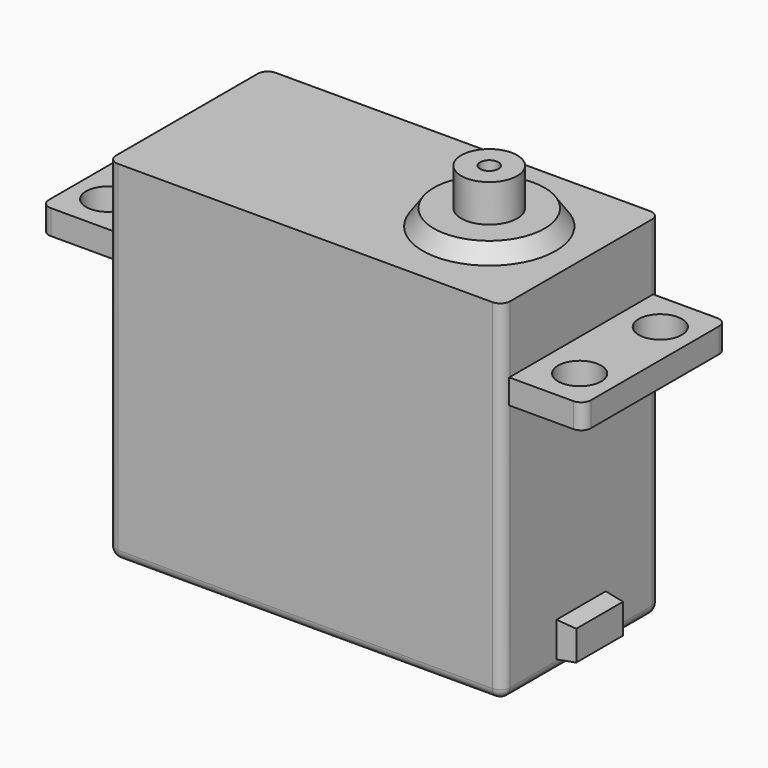
from build123d import *

# Parameters (mm, degrees)
F0_W           = 40.64
F0_H           = 20.32
F1_DEPTH       = 36.068
F2_W           = 6.35
F2_H           = 3.6068
F4_W           = 6.0198
F4_H           = 3.0734
F7_R           = 2.2225
F8_DEPTH       = 2.54
F9_R           = 6.858
F11_R          = 5.7023
F13_T1_DEPTH   = 38.608
F13_T3_DEPTH   = 18.288
F13_S7_W       = 1.016
F13_S7_H       = 1.016
F13_T8_DEPTH   = 1.016
F13_S13_W      = 1.016
F13_S13_H      = 1.016
F13_T14_DEPTH  = 1.016
F13_S19_W      = 1.016
F13_S19_H      = 1.016
F13_T20_DEPTH  = 1.016
F13_S25_W      = 1.016
F13_S25_H      = 1.016
F13_T26_DEPTH  = 1.016
F13_T32_DEPTH  = 37.592
F13_T38_DEPTH  = 37.592
F13_T44_DEPTH  = 37.592
F13_T51_DEPTH  = 37.592
F13_T57_DEPTH  = 37.592
F13_T63_DEPTH  = 37.592
F13_T69_DEPTH  = 37.592
F13_T75_DEPTH  = 37.592
F13_T82_DEPTH  = 37.592
F13_T88_DEPTH  = 37.592
F13_T94_DEPTH  = 37.592
F13_T100_DEPTH = 37.592
F13_T106_DEPTH = 37.592
F13_T113_DEPTH = 37.592
F13_T119_DEPTH = 37.592
F13_T125_DEPTH = 37.592
F13_T131_DEPTH = 37.592
F13_T137_DEPTH = 37.592
F13_T144_DEPTH = 37.592
F13_T150_DEPTH = 37.592
F14_R          = 2.8829
F14_R_2        = 0.9398
F15_DEPTH      = 3.8608


# Not quite as in the source:
# - a fillet or chamfer that OpenCascade refuses, or shapes differently, is made with other operations: its cross-section is extruded or revolved along the edge and cut away or added


with BuildPart() as f1:
    # F0 (on Top) → F1 (new body)
    with BuildSketch(Plane.XY):
        Rectangle(F0_W, F0_H)
    extrude(amount=F1_DEPTH)

    # F2 (on face) → F5 section 0
    with BuildSketch(Plane.YZ.offset(20.32)):
        with Locations((0, 2.9464)):
            Rectangle(F2_W, F2_H)
    # F4 (on offset) → F5 section 1
    with BuildSketch(Plane.YZ.offset(22.225)):
        with Locations((0, 2.9464)):
            Rectangle(F4_W, F4_H)
    loft()

    # F7 (on offset) → F8 (join)
    with BuildSketch(Plane.XY.offset(29.21)):
        with BuildLine():
            ThreePointArc((-27.94, -8.255), (-27.6424204897, -8.9734204897), (-26.924, -9.271))
            Line((-26.924, -9.271), (-20.32, -9.271))
            Line((-20.32, -9.271), (-20.32, 9.271))
            Line((-20.32, 9.271), (-26.924, 9.271))
            ThreePointArc((-26.924, 9.271), (-27.6424204897, 8.9734204897), (-27.94, 8.255))
            Line((-27.94, 8.255), (-27.94, -8.255))
        make_face()
        with Locations((-24.3205, -5.1943)):
            Circle(F7_R, mode=Mode.SUBTRACT)
        with Locations((-24.3205, 5.1943)):
            Circle(F7_R, mode=Mode.SUBTRACT)
        with BuildLine():
            ThreePointArc((27.94, 8.255), (27.6424204897, 8.9734204897), (26.924, 9.271))
            Line((26.924, 9.271), (20.32, 9.271))
            Line((20.32, 9.271), (20.32, -9.271))
            Line((20.32, -9.271), (26.924, -9.271))
            ThreePointArc((26.924, -9.271), (27.6424204897, -8.9734204897), (27.94, -8.255))
            Line((27.94, -8.255), (27.94, 8.255))
        make_face()
        with Locations((24.3205, -5.1943)):
            Circle(F7_R, mode=Mode.SUBTRACT)
        with Locations((24.3205, 5.1943)):
            Circle(F7_R, mode=Mode.SUBTRACT)
    extrude(amount=-F8_DEPTH)

    # F9 (on face) → F12 section 0
    with BuildSketch(Plane.XY.offset(36.068)):
        with Locations((10.8458, 0)):
            Circle(F9_R)
    # F11 (on offset) → F12 section 1
    with BuildSketch(Plane.XY.offset(37.719)):
        with Locations((10.8458, 0)):
            Circle(F11_R)
    loft()

    # F13: fillet of radius 1.016 on 8 edges, made by hand

    # F13_s2 → F13_t1 (cut)
    with BuildSketch(Plane.YZ.offset(-19.304)):
        with BuildLine():
            ThreePointArc((-10.16, 1.016), (-9.8624204897, 0.2975795103), (-9.144, 0))
            Line((-9.144, 0), (-10.16, 0))
            Line((-10.16, 0), (-10.16, 1.016))
        make_face()
        with BuildLine():
            ThreePointArc((9.144, 0), (9.8624204897, 0.2975795103), (10.16, 1.016))
            Line((10.16, 1.016), (10.16, 0))
            Line((10.16, 0), (9.144, 0))
        make_face()
    extrude(amount=F13_T1_DEPTH, mode=Mode.SUBTRACT)

    # F13_s4 → F13_t3 (cut)
    with BuildSketch(Plane.XZ.offset(-9.144)):
        with BuildLine():
            ThreePointArc((20.32, 1.016), (20.0224204897, 0.2975795103), (19.304, 0))
            Line((19.304, 0), (20.32, 0))
            Line((20.32, 0), (20.32, 1.016))
        make_face()
        with BuildLine():
            ThreePointArc((-19.304, 0), (-20.0224204897, 0.2975795103), (-20.32, 1.016))
            Line((-20.32, 1.016), (-20.32, 0))
            Line((-20.32, 0), (-19.304, 0))
        make_face()
    extrude(amount=F13_T3_DEPTH, mode=Mode.SUBTRACT)


with BuildPart() as f13_tool6:
    # F13_s7 → F13_t8 (new body)
    with BuildSketch(Plane.YZ.offset(19.304)):
        with Locations((-9.652, 0.508)):
            Rectangle(F13_S7_W, F13_S7_H)
    extrude(amount=F13_T8_DEPTH)

    # F13_s9 → F13_t10 (revolve, cut)
    with BuildSketch(Plane(origin=(19.304, -9.144, 1.016), x_dir=(0, 0.7071067812, 0.7071067812), z_dir=(0, 0.7071067812, -0.7071067812))):
        with BuildLine():
            ThreePointArc((0, -1.016), (1.016, 0), (0, 1.016))
            Line((0, 1.016), (0, -1.016))
        make_face()
    revolve(axis=Axis((19.304, -9.144, 1.016), (1, 0, 0)), mode=Mode.SUBTRACT)


with BuildPart() as f1_1:
    add(f1.part)

    # F13_t5: cut F13_tool6
    add(f13_tool6.part, mode=Mode.SUBTRACT)


with BuildPart() as f13_tool12:
    # F13_s13 → F13_t14 (new body)
    with BuildSketch(Plane.YZ.offset(19.304)):
        with Locations((9.652, 0.508)):
            Rectangle(F13_S13_W, F13_S13_H)
    extrude(amount=F13_T14_DEPTH)

    # F13_s15 → F13_t16 (revolve, cut)
    with BuildSketch(Plane(origin=(19.304, 9.144, 1.016), x_dir=(0, -0.7071067812, 0.7071067812), z_dir=(0, 0.7071067812, 0.7071067812))):
        with BuildLine():
            ThreePointArc((0, -1.016), (1.016, 0), (0, 1.016))
            Line((0, 1.016), (0, -1.016))
        make_face()
    revolve(axis=Axis((19.304, 9.144, 1.016), (1, 0, 0)), mode=Mode.SUBTRACT)


with BuildPart() as f1_2:
    add(f1_1.part)

    # F13_t11: cut F13_tool12
    add(f13_tool12.part, mode=Mode.SUBTRACT)


with BuildPart() as f13_tool18:
    # F13_s19 → F13_t20 (new body)
    with BuildSketch(Plane.XY.offset(1.016)):
        with Locations((-19.812, 9.652)):
            Rectangle(F13_S19_W, F13_S19_H)
    extrude(amount=-F13_T20_DEPTH)

    # F13_s21 → F13_t22 (revolve, cut)
    with BuildSketch(Plane(origin=(-19.304, 9.144, 1.016), x_dir=(0.7071067812, -0.7071067812, 0), z_dir=(0.7071067812, 0.7071067812, 0))):
        with BuildLine():
            ThreePointArc((0, -1.016), (1.016, 0), (0, 1.016))
            Line((0, 1.016), (0, -1.016))
        make_face()
    revolve(axis=Axis((-19.304, 9.144, 1.016), (0, 0, -1)), mode=Mode.SUBTRACT)


with BuildPart() as f1_3:
    add(f1_2.part)

    # F13_t17: cut F13_tool18
    add(f13_tool18.part, mode=Mode.SUBTRACT)


with BuildPart() as f13_tool24:
    # F13_s25 → F13_t26 (new body)
    with BuildSketch(Plane.XZ.offset(9.144)):
        with Locations((-19.812, 0.508)):
            Rectangle(F13_S25_W, F13_S25_H)
    extrude(amount=F13_T26_DEPTH)

    # F13_s27 → F13_t28 (revolve, cut)
    with BuildSketch(Plane(origin=(-19.304, -9.144, 1.016), x_dir=(0.7071067812, 0, 0.7071067812), z_dir=(0.7071067812, 0, -0.7071067812))):
        with BuildLine():
            ThreePointArc((0, -1.016), (1.016, 0), (0, 1.016))
            Line((0, 1.016), (0, -1.016))
        make_face()
    revolve(axis=Axis((-19.304, -9.144, 1.016), (0, -1, 0)), mode=Mode.SUBTRACT)


with BuildPart() as f1_4:
    add(f1_3.part)

    # F13_t23: cut F13_tool24
    add(f13_tool24.part, mode=Mode.SUBTRACT)


with BuildPart() as f13_tool30:
    # F13_s31 → F13_t32 (new body)
    with BuildSketch(Plane.XY.offset(1.016)):
        with BuildLine():
            ThreePointArc((20.32, -9.144), (20.0224204897, -9.8624204897), (19.304, -10.16))
            Line((19.304, -10.16), (20.32, -10.16))
            Line((20.32, -10.16), (20.32, -9.144))
        make_face()
    extrude(amount=F13_T32_DEPTH)

    split(bisect_by=Plane.XY.offset(26.67), keep=Keep.BOTTOM)

    split(bisect_by=Plane.XZ.offset(9.271), keep=Keep.BOTTOM)


with BuildPart() as f1_5:
    add(f1_4.part)

    # F13_t29: cut F13_tool30
    add(f13_tool30.part, mode=Mode.SUBTRACT)


with BuildPart() as f13_tool36:
    # F13_s37 → F13_t38 (new body)
    with BuildSketch(Plane.XY.offset(1.016)):
        with BuildLine():
            ThreePointArc((20.32, -9.144), (20.0224204897, -9.8624204897), (19.304, -10.16))
            Line((19.304, -10.16), (20.32, -10.16))
            Line((20.32, -10.16), (20.32, -9.144))
        make_face()
    extrude(amount=F13_T38_DEPTH)

    split(bisect_by=Plane.XY.offset(26.67), keep=Keep.BOTTOM)

    split(bisect_by=Plane.XZ.offset(9.271), keep=Keep.TOP)


with BuildPart() as f1_6:
    add(f1_5.part)

    # F13_t35: cut F13_tool36
    add(f13_tool36.part, mode=Mode.SUBTRACT)


with BuildPart() as f13_tool42:
    # F13_s43 → F13_t44 (new body)
    with BuildSketch(Plane.XY.offset(1.016)):
        with BuildLine():
            ThreePointArc((20.32, -9.144), (20.0224204897, -9.8624204897), (19.304, -10.16))
            Line((19.304, -10.16), (20.32, -10.16))
            Line((20.32, -10.16), (20.32, -9.144))
        make_face()
    extrude(amount=F13_T44_DEPTH)

    split(bisect_by=Plane.XY.offset(26.67), keep=Keep.TOP)

    split(bisect_by=Plane.XZ.offset(9.271), keep=Keep.TOP)

    split(bisect_by=Plane.XY.offset(29.21), keep=Keep.BOTTOM)


with BuildPart() as f1_7:
    add(f1_6.part)

    # F13_t41: cut F13_tool42
    add(f13_tool42.part, mode=Mode.SUBTRACT)


with BuildPart() as f13_tool49:
    # F13_s50 → F13_t51 (new body)
    with BuildSketch(Plane.XY.offset(1.016)):
        with BuildLine():
            ThreePointArc((20.32, -9.144), (20.0224204897, -9.8624204897), (19.304, -10.16))
            Line((19.304, -10.16), (20.32, -10.16))
            Line((20.32, -10.16), (20.32, -9.144))
        make_face()
    extrude(amount=F13_T51_DEPTH)

    split(bisect_by=Plane.XZ.offset(9.271), keep=Keep.BOTTOM)

    split(bisect_by=Plane.XY.offset(29.21), keep=Keep.TOP)


with BuildPart() as f1_8:
    add(f1_7.part)

    # F13_t48: cut F13_tool49
    add(f13_tool49.part, mode=Mode.SUBTRACT)


with BuildPart() as f13_tool55:
    # F13_s56 → F13_t57 (new body)
    with BuildSketch(Plane.XY.offset(1.016)):
        with BuildLine():
            ThreePointArc((20.32, -9.144), (20.0224204897, -9.8624204897), (19.304, -10.16))
            Line((19.304, -10.16), (20.32, -10.16))
            Line((20.32, -10.16), (20.32, -9.144))
        make_face()
    extrude(amount=F13_T57_DEPTH)

    split(bisect_by=Plane.XZ.offset(9.271), keep=Keep.TOP)

    split(bisect_by=Plane.XY.offset(29.21), keep=Keep.TOP)


with BuildPart() as f1_9:
    add(f1_8.part)

    # F13_t54: cut F13_tool55
    add(f13_tool55.part, mode=Mode.SUBTRACT)


with BuildPart() as f13_tool61:
    # F13_s62 → F13_t63 (new body)
    with BuildSketch(Plane.XY.offset(1.016)):
        with BuildLine():
            ThreePointArc((20.32, 9.144), (20.0224204897, 9.8624204897), (19.304, 10.16))
            Line((19.304, 10.16), (20.32, 10.16))
            Line((20.32, 10.16), (20.32, 9.144))
        make_face()
    extrude(amount=F13_T63_DEPTH)

    split(bisect_by=Plane.XZ.offset(-9.271), keep=Keep.TOP)

    split(bisect_by=Plane.XY.offset(26.67), keep=Keep.BOTTOM)


with BuildPart() as f1_10:
    add(f1_9.part)

    # F13_t60: cut F13_tool61
    add(f13_tool61.part, mode=Mode.SUBTRACT)


with BuildPart() as f13_tool67:
    # F13_s68 → F13_t69 (new body)
    with BuildSketch(Plane.XY.offset(1.016)):
        with BuildLine():
            ThreePointArc((20.32, 9.144), (20.0224204897, 9.8624204897), (19.304, 10.16))
            Line((19.304, 10.16), (20.32, 10.16))
            Line((20.32, 10.16), (20.32, 9.144))
        make_face()
    extrude(amount=F13_T69_DEPTH)

    split(bisect_by=Plane.XZ.offset(-9.271), keep=Keep.BOTTOM)

    split(bisect_by=Plane.XY.offset(26.67), keep=Keep.BOTTOM)


with BuildPart() as f1_11:
    add(f1_10.part)

    # F13_t66: cut F13_tool67
    add(f13_tool67.part, mode=Mode.SUBTRACT)


with BuildPart() as f13_tool73:
    # F13_s74 → F13_t75 (new body)
    with BuildSketch(Plane.XY.offset(1.016)):
        with BuildLine():
            ThreePointArc((20.32, 9.144), (20.0224204897, 9.8624204897), (19.304, 10.16))
            Line((19.304, 10.16), (20.32, 10.16))
            Line((20.32, 10.16), (20.32, 9.144))
        make_face()
    extrude(amount=F13_T75_DEPTH)

    split(bisect_by=Plane.XZ.offset(-9.271), keep=Keep.BOTTOM)

    split(bisect_by=Plane.XY.offset(26.67), keep=Keep.TOP)

    split(bisect_by=Plane.XY.offset(29.21), keep=Keep.BOTTOM)


with BuildPart() as f1_12:
    add(f1_11.part)

    # F13_t72: cut F13_tool73
    add(f13_tool73.part, mode=Mode.SUBTRACT)


with BuildPart() as f13_tool80:
    # F13_s81 → F13_t82 (new body)
    with BuildSketch(Plane.XY.offset(1.016)):
        with BuildLine():
            ThreePointArc((20.32, 9.144), (20.0224204897, 9.8624204897), (19.304, 10.16))
            Line((19.304, 10.16), (20.32, 10.16))
            Line((20.32, 10.16), (20.32, 9.144))
        make_face()
    extrude(amount=F13_T82_DEPTH)

    split(bisect_by=Plane.XZ.offset(-9.271), keep=Keep.TOP)

    split(bisect_by=Plane.XY.offset(29.21), keep=Keep.TOP)


with BuildPart() as f1_13:
    add(f1_12.part)

    # F13_t79: cut F13_tool80
    add(f13_tool80.part, mode=Mode.SUBTRACT)


with BuildPart() as f13_tool86:
    # F13_s87 → F13_t88 (new body)
    with BuildSketch(Plane.XY.offset(1.016)):
        with BuildLine():
            ThreePointArc((20.32, 9.144), (20.0224204897, 9.8624204897), (19.304, 10.16))
            Line((19.304, 10.16), (20.32, 10.16))
            Line((20.32, 10.16), (20.32, 9.144))
        make_face()
    extrude(amount=F13_T88_DEPTH)

    split(bisect_by=Plane.XZ.offset(-9.271), keep=Keep.BOTTOM)

    split(bisect_by=Plane.XY.offset(29.21), keep=Keep.TOP)


with BuildPart() as f1_14:
    add(f1_13.part)

    # F13_t85: cut F13_tool86
    add(f13_tool86.part, mode=Mode.SUBTRACT)


with BuildPart() as f13_tool92:
    # F13_s93 → F13_t94 (new body)
    with BuildSketch(Plane.XY.offset(1.016)):
        with BuildLine():
            ThreePointArc((-19.304, 10.16), (-20.0224204897, 9.8624204897), (-20.32, 9.144))
            Line((-20.32, 9.144), (-20.32, 10.16))
            Line((-20.32, 10.16), (-19.304, 10.16))
        make_face()
    extrude(amount=F13_T94_DEPTH)

    split(bisect_by=Plane.XY.offset(26.67), keep=Keep.BOTTOM)

    split(bisect_by=Plane.XZ.offset(-9.271), keep=Keep.BOTTOM)


with BuildPart() as f1_15:
    add(f1_14.part)

    # F13_t91: cut F13_tool92
    add(f13_tool92.part, mode=Mode.SUBTRACT)


with BuildPart() as f13_tool98:
    # F13_s99 → F13_t100 (new body)
    with BuildSketch(Plane.XY.offset(1.016)):
        with BuildLine():
            ThreePointArc((-19.304, 10.16), (-20.0224204897, 9.8624204897), (-20.32, 9.144))
            Line((-20.32, 9.144), (-20.32, 10.16))
            Line((-20.32, 10.16), (-19.304, 10.16))
        make_face()
    extrude(amount=F13_T100_DEPTH)

    split(bisect_by=Plane.XY.offset(26.67), keep=Keep.BOTTOM)

    split(bisect_by=Plane.XZ.offset(-9.271), keep=Keep.TOP)


with BuildPart() as f1_16:
    add(f1_15.part)

    # F13_t97: cut F13_tool98
    add(f13_tool98.part, mode=Mode.SUBTRACT)


with BuildPart() as f13_tool104:
    # F13_s105 → F13_t106 (new body)
    with BuildSketch(Plane.XY.offset(1.016)):
        with BuildLine():
            ThreePointArc((-19.304, 10.16), (-20.0224204897, 9.8624204897), (-20.32, 9.144))
            Line((-20.32, 9.144), (-20.32, 10.16))
            Line((-20.32, 10.16), (-19.304, 10.16))
        make_face()
    extrude(amount=F13_T106_DEPTH)

    split(bisect_by=Plane.XY.offset(26.67), keep=Keep.TOP)

    split(bisect_by=Plane.XZ.offset(-9.271), keep=Keep.BOTTOM)

    split(bisect_by=Plane.XY.offset(29.21), keep=Keep.BOTTOM)


with BuildPart() as f1_17:
    add(f1_16.part)

    # F13_t103: cut F13_tool104
    add(f13_tool104.part, mode=Mode.SUBTRACT)


with BuildPart() as f13_tool111:
    # F13_s112 → F13_t113 (new body)
    with BuildSketch(Plane.XY.offset(1.016)):
        with BuildLine():
            ThreePointArc((-19.304, 10.16), (-20.0224204897, 9.8624204897), (-20.32, 9.144))
            Line((-20.32, 9.144), (-20.32, 10.16))
            Line((-20.32, 10.16), (-19.304, 10.16))
        make_face()
    extrude(amount=F13_T113_DEPTH)

    split(bisect_by=Plane.XZ.offset(-9.271), keep=Keep.BOTTOM)

    split(bisect_by=Plane.XY.offset(29.21), keep=Keep.TOP)


with BuildPart() as f1_18:
    add(f1_17.part)

    # F13_t110: cut F13_tool111
    add(f13_tool111.part, mode=Mode.SUBTRACT)


with BuildPart() as f13_tool117:
    # F13_s118 → F13_t119 (new body)
    with BuildSketch(Plane.XY.offset(1.016)):
        with BuildLine():
            ThreePointArc((-19.304, 10.16), (-20.0224204897, 9.8624204897), (-20.32, 9.144))
            Line((-20.32, 9.144), (-20.32, 10.16))
            Line((-20.32, 10.16), (-19.304, 10.16))
        make_face()
    extrude(amount=F13_T119_DEPTH)

    split(bisect_by=Plane.XZ.offset(-9.271), keep=Keep.TOP)

    split(bisect_by=Plane.XY.offset(29.21), keep=Keep.TOP)


with BuildPart() as f1_19:
    add(f1_18.part)

    # F13_t116: cut F13_tool117
    add(f13_tool117.part, mode=Mode.SUBTRACT)


with BuildPart() as f13_tool123:
    # F13_s124 → F13_t125 (new body)
    with BuildSketch(Plane.XY.offset(1.016)):
        with BuildLine():
            ThreePointArc((-19.304, -10.16), (-20.0224204897, -9.8624204897), (-20.32, -9.144))
            Line((-20.32, -9.144), (-20.32, -10.16))
            Line((-20.32, -10.16), (-19.304, -10.16))
        make_face()
    extrude(amount=F13_T125_DEPTH)

    split(bisect_by=Plane.XZ.offset(9.271), keep=Keep.TOP)

    split(bisect_by=Plane.XY.offset(26.67), keep=Keep.BOTTOM)


with BuildPart() as f1_20:
    add(f1_19.part)

    # F13_t122: cut F13_tool123
    add(f13_tool123.part, mode=Mode.SUBTRACT)


with BuildPart() as f13_tool129:
    # F13_s130 → F13_t131 (new body)
    with BuildSketch(Plane.XY.offset(1.016)):
        with BuildLine():
            ThreePointArc((-19.304, -10.16), (-20.0224204897, -9.8624204897), (-20.32, -9.144))
            Line((-20.32, -9.144), (-20.32, -10.16))
            Line((-20.32, -10.16), (-19.304, -10.16))
        make_face()
    extrude(amount=F13_T131_DEPTH)

    split(bisect_by=Plane.XZ.offset(9.271), keep=Keep.BOTTOM)

    split(bisect_by=Plane.XY.offset(26.67), keep=Keep.BOTTOM)


with BuildPart() as f1_21:
    add(f1_20.part)

    # F13_t128: cut F13_tool129
    add(f13_tool129.part, mode=Mode.SUBTRACT)


with BuildPart() as f13_tool135:
    # F13_s136 → F13_t137 (new body)
    with BuildSketch(Plane.XY.offset(1.016)):
        with BuildLine():
            ThreePointArc((-19.304, -10.16), (-20.0224204897, -9.8624204897), (-20.32, -9.144))
            Line((-20.32, -9.144), (-20.32, -10.16))
            Line((-20.32, -10.16), (-19.304, -10.16))
        make_face()
    extrude(amount=F13_T137_DEPTH)

    split(bisect_by=Plane.XZ.offset(9.271), keep=Keep.TOP)

    split(bisect_by=Plane.XY.offset(26.67), keep=Keep.TOP)

    split(bisect_by=Plane.XY.offset(29.21), keep=Keep.BOTTOM)


with BuildPart() as f1_22:
    add(f1_21.part)

    # F13_t134: cut F13_tool135
    add(f13_tool135.part, mode=Mode.SUBTRACT)


with BuildPart() as f13_tool142:
    # F13_s143 → F13_t144 (new body)
    with BuildSketch(Plane.XY.offset(1.016)):
        with BuildLine():
            ThreePointArc((-19.304, -10.16), (-20.0224204897, -9.8624204897), (-20.32, -9.144))
            Line((-20.32, -9.144), (-20.32, -10.16))
            Line((-20.32, -10.16), (-19.304, -10.16))
        make_face()
    extrude(amount=F13_T144_DEPTH)

    split(bisect_by=Plane.XZ.offset(9.271), keep=Keep.TOP)

    split(bisect_by=Plane.XY.offset(29.21), keep=Keep.TOP)


with BuildPart() as f1_23:
    add(f1_22.part)

    # F13_t141: cut F13_tool142
    add(f13_tool142.part, mode=Mode.SUBTRACT)


with BuildPart() as f13_tool148:
    # F13_s149 → F13_t150 (new body)
    with BuildSketch(Plane.XY.offset(1.016)):
        with BuildLine():
            ThreePointArc((-19.304, -10.16), (-20.0224204897, -9.8624204897), (-20.32, -9.144))
            Line((-20.32, -9.144), (-20.32, -10.16))
            Line((-20.32, -10.16), (-19.304, -10.16))
        make_face()
    extrude(amount=F13_T150_DEPTH)

    split(bisect_by=Plane.XZ.offset(9.271), keep=Keep.BOTTOM)

    split(bisect_by=Plane.XY.offset(29.21), keep=Keep.TOP)


with BuildPart() as f1_24:
    add(f1_23.part)

    # F13_t147: cut F13_tool148
    add(f13_tool148.part, mode=Mode.SUBTRACT)

    # F14 (on face) → F15 (join)
    with BuildSketch(Plane.XY.offset(37.719)):
        with Locations((10.8458, 0)):
            Circle(F14_R)
        with Locations((10.8458, 0)):
            Circle(F14_R_2, mode=Mode.SUBTRACT)
    extrude(amount=F15_DEPTH)


solid = f1_24.part
